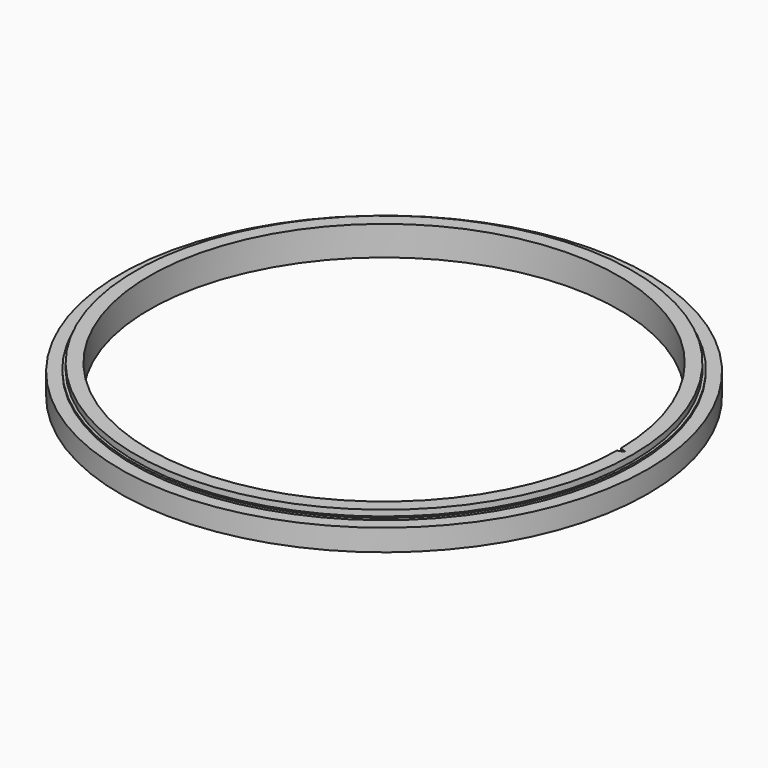
from build123d import *

# Parameters (mm, degrees)
F0_R        = 67
F0_R_2      = 59.6
F1_DEPTH    = 3.75
F2_R        = 63.875
F2_R_2      = 63.125
F3_DEPTH    = 1.5
F3_FACE_R   = 67
F3_FACE_R_2 = 63.875
F4_DEPTH    = 2
F4_TAPER    = -3
F7_DEPTH    = 6.5
F7_TAPER    = -3


# Not quite as in the source:
# - a feature of the source that left no trace in its solid (it failed there, or was rolled back) is left out


with BuildPart() as f1:
    # F0 (on Top) → F1 (new body, symmetric)
    with BuildSketch(Plane.XY):
        Circle(F0_R)
        Circle(F0_R_2, mode=Mode.SUBTRACT)
    extrude(amount=F1_DEPTH, both=True)

    # F2 (on face) → F3 (cut)
    with BuildSketch(Plane.XY.offset(3.75)):
        Circle(F2_R)
        Circle(F2_R_2, mode=Mode.SUBTRACT)
    extrude(amount=-F3_DEPTH, mode=Mode.SUBTRACT)

    # F3_face (on face) → F4 (cut)
    with BuildSketch(Plane.XY.offset(3.75)):
        Circle(F3_FACE_R)
        Circle(F3_FACE_R_2, mode=Mode.SUBTRACT)
    extrude(amount=-F4_DEPTH, taper=F4_TAPER, mode=Mode.SUBTRACT)

    # F6 (on face) → F7 (cut)
    with BuildSketch(Plane.XY.offset(3.75)):
        Polygon((61, 0.15), (59.4, 0.675), (59.4, -0.675), (61, -0.15), align=None)
    extrude(amount=-F7_DEPTH, taper=F7_TAPER, mode=Mode.SUBTRACT)


solid = f1.part
